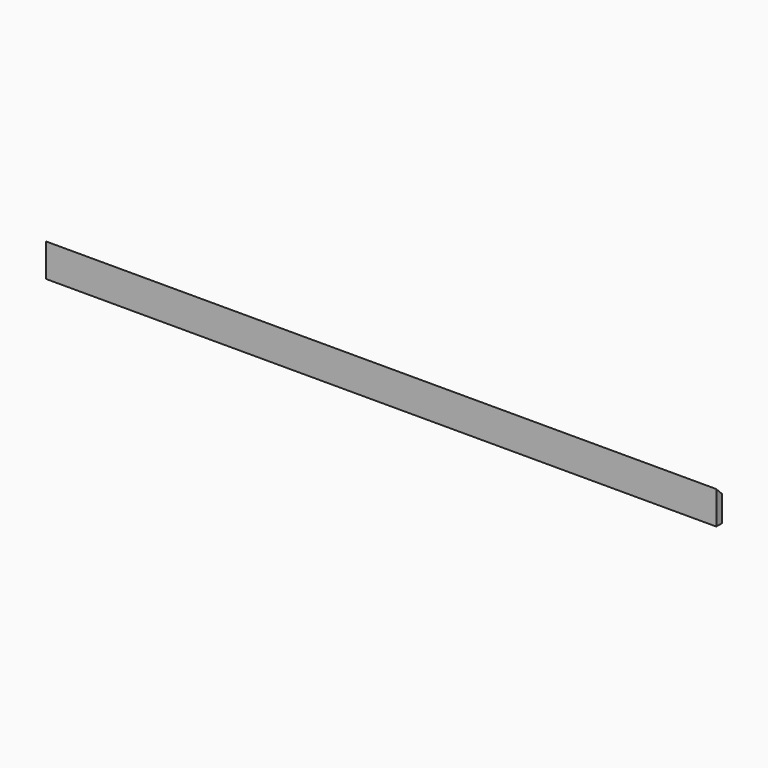
from build123d import *

# Parameters (mm, degrees)
F0_W     = 1801.5966
F0_H     = 88.9
F1_DEPTH = 9.525
F2_SIZE  = 19.04999


# Not quite as in the source:
# - a fillet or chamfer is up to 0.001 mm smaller than in the source, because OpenCascade refuses the exact size


with BuildPart() as f1:
    # F0 (on Front) → F1 (new body, symmetric)
    with BuildSketch(Plane.XZ):
        Rectangle(F0_W, F0_H)
    extrude(amount=F1_DEPTH, both=True)

    # F2 (size 19.05 in the source; OpenCascade refuses exactly that, so slightly less here)
    f2_edges = [f1.edges().sort_by_distance(p)[0] for p in [
        (0, 9.525, 44.45),
    ]]
    chamfer(f2_edges, length=F2_SIZE)


solid = f1.part
